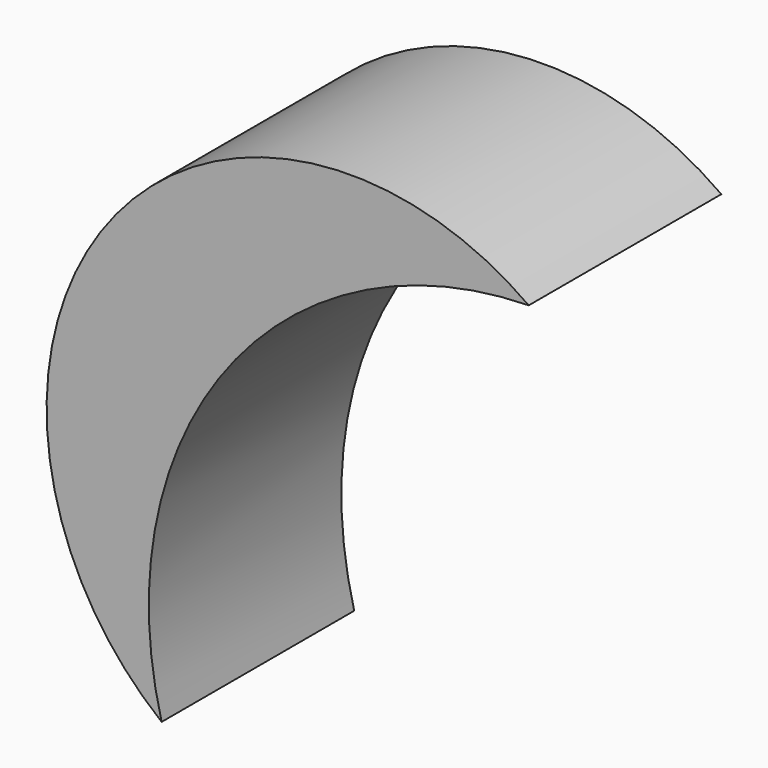
from build123d import *

# Parameters (mm, degrees)
F1_DEPTH = 25.4
F2_DEPTH = 37.2688174248


with BuildPart() as f1:
    # F0 (on Front) → F1 (new body)
    with BuildSketch(Plane.XZ):
        with BuildLine():
            ThreePointArc((-104.9915319686, 14.58820215), (-87.9650318686, 101.10781826), (-9.4045125971, 141.155171347))
            ThreePointArc((-9.4045125971, 141.155171347), (-118.917828322, 124.4842613633), (-104.9915319686, 14.58820215))
        make_face()
    extrude(amount=F1_DEPTH)

    # F2 (add): a face of the model
    f2_faces = [f1.faces().sort_by_distance(p)[0] for p in [
        (-94.2711114093, 0, 105.8703510997),
    ]]
    extrude(f2_faces, amount=F2_DEPTH)


solid = f1.part
